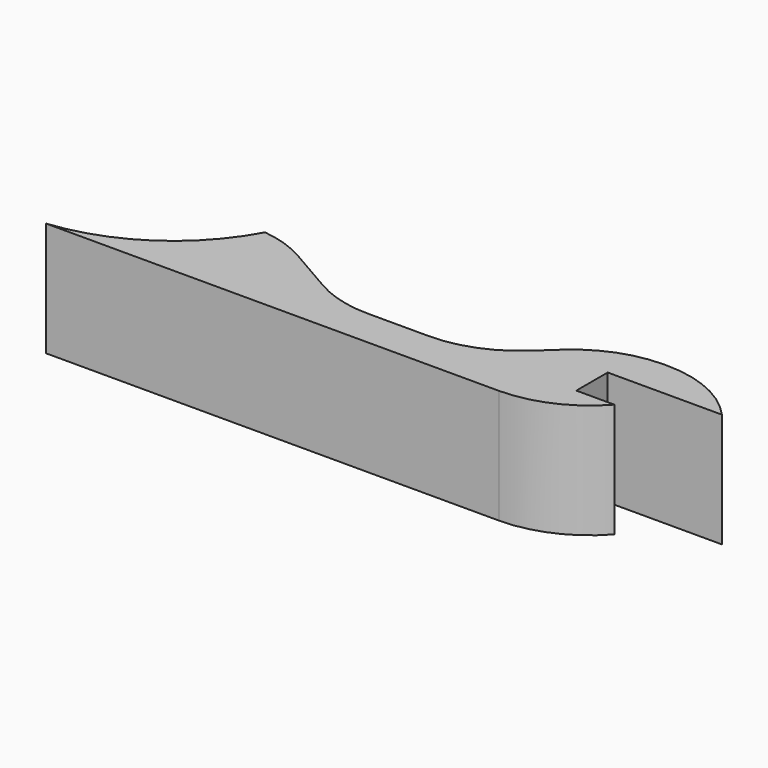
from build123d import *

# Parameters (mm, degrees)
F1_DEPTH    = 7.62
F2_T1_DEPTH = 7.62
F2_T3_DEPTH = 7.62
F2_T5_DEPTH = 22.4683303368
F2_T7_DEPTH = 17.3475037725
F3_T1_DEPTH = 36.0180633142


# Not quite as in the source:
# - a fillet or chamfer that OpenCascade refuses, or shapes differently, is made with other operations: its cross-section is extruded or revolved along the edge and cut away or added


with BuildPart() as f1:
    # F0 (on Top) → F1 (new body)
    with BuildSketch(Plane.XY):
        with BuildLine():
            Line((-9.525, 0), (0, 0))
            Line((0, 0), (23.8125, 0))
            Line((23.8125, 0), (26.3525, 0))
            Line((26.3525, 0), (26.3525, 2.54))
            Line((26.3525, 2.54), (23.8125, 2.54))
            Line((23.8125, 2.54), (23.8125, 5.1562))
            Line((23.8125, 5.1562), (31.4325, 5.1562))
            Line((31.4325, 5.1562), (31.4325, 7.6962))
            Line((31.4325, 7.6962), (22.5425, 7.6962))
            Line((22.5425, 7.6962), (16.9319740389, 2.54))
            Line((16.9319740389, 2.54), (7.8691135768, 2.54))
            Line((7.8691135768, 2.54), (1.27, 6.35))
            Line((1.27, 6.35), (0, 6.35))
            ThreePointArc((0, 6.35), (-3.9738865155, 1.9920797732), (-9.525, 0))
        make_face()
    extrude(amount=F1_DEPTH)

    # F2: fillet of radius 7.62 on 4 edges, made by hand

    # F2_s2 → F2_t1 (join)
    with BuildSketch(Plane.XY):
        with BuildLine():
            ThreePointArc((13.9623079716, 2.54), (16.729273112, 3.0601194438), (19.1185079716, 4.5494740389))
            Line((19.1185079716, 4.5494740389), (16.9319740389, 2.54))
            Line((16.9319740389, 2.54), (13.9623079716, 2.54))
        make_face()
    extrude(amount=F2_T1_DEPTH)

    # F2_s4 → F2_t3 (join)
    with BuildSketch(Plane.XY):
        with BuildLine():
            ThreePointArc((9.9108864232, 2.54), (7.9386852995, 2.7996452037), (6.1008864232, 3.5608864232))
            Line((6.1008864232, 3.5608864232), (7.8691135768, 2.54))
            Line((7.8691135768, 2.54), (9.9108864232, 2.54))
        make_face()
    extrude(amount=F2_T3_DEPTH)

    # F2_s6 → F2_t5 (cut)
    with BuildSketch(Plane.XY.offset(-7.4241651684)):
        with BuildLine():
            ThreePointArc((25.5121660674, 7.6962), (22.7452009269, 7.1760805562), (20.3559660674, 5.6867259611))
            Line((20.3559660674, 5.6867259611), (22.5425, 7.6962))
            Line((22.5425, 7.6962), (25.5121660674, 7.6962))
        make_face()
    extrude(amount=F2_T5_DEPTH, mode=Mode.SUBTRACT)

    # F2_s8 → F2_t7 (cut)
    with BuildSketch(Plane.XY.offset(-4.8637518862)):
        with BuildLine():
            ThreePointArc((0, 6.35), (1.5275951478, 6.0160183482), (2.9548530765, 5.3772496228))
            Line((2.9548530765, 5.3772496228), (1.27, 6.35))
            Line((1.27, 6.35), (0, 6.35))
        make_face()
    extrude(amount=F2_T7_DEPTH, mode=Mode.SUBTRACT)

    # F3: fillet of radius 7.62 on 2 edges, made by hand

    # F3_s2 → F3_t1 (cut)
    with BuildSketch(Plane.XY.offset(-14.1990316571)):
        with BuildLine():
            ThreePointArc((25.7528873372, 7.6962), (28.8637393105, 7.0322764803), (31.4325, 5.1562))
            Line((31.4325, 5.1562), (31.4325, 7.6962))
            Line((31.4325, 7.6962), (25.7528873372, 7.6962))
        make_face()
        with BuildLine():
            ThreePointArc((26.3525, 2.54), (23.7837393105, 0.6639235197), (20.6728873372, 0))
            Line((20.6728873372, 0), (26.3525, 0))
            Line((26.3525, 0), (26.3525, 2.54))
        make_face()
    extrude(amount=F3_T1_DEPTH, mode=Mode.SUBTRACT)


solid = f1.part
